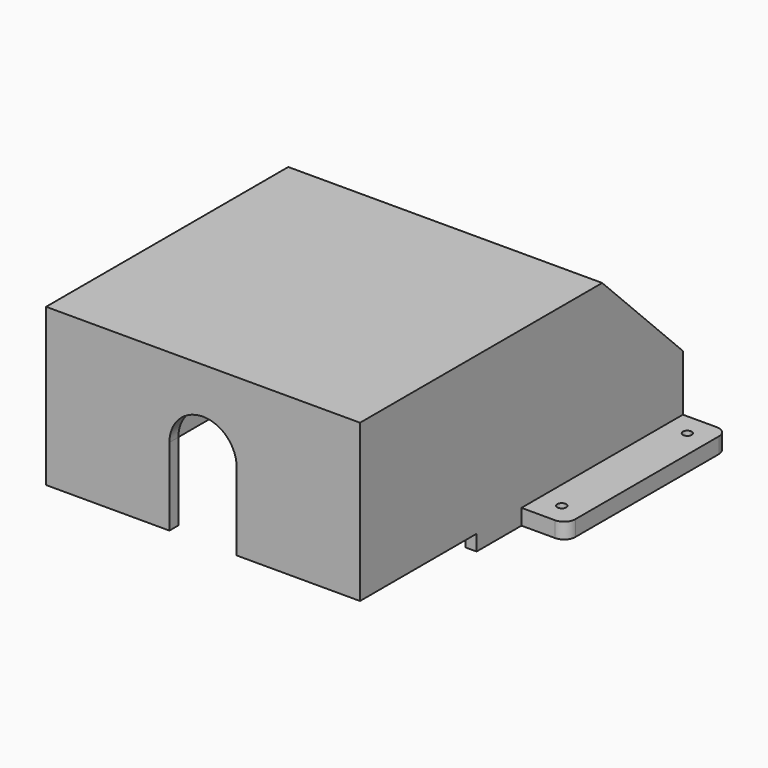
from build123d import *

# Parameters (mm, degrees)
F0_W      = 140
F0_H      = 180
F1_DEPTH  = 70
F2_W      = 130
F2_H      = 170
F3_DEPTH  = 65
F4_SIZE   = 45
F5_W      = 30
F5_H      = 49.6265143156
F6_DEPTH  = 25
F7_R      = 14.99999
F9_DEPTH  = 7
F10_W     = 59.1894394159
F10_H     = 26.9657306075
F11_DEPTH = 25
F12_W     = 90
F12_H     = 7
F13_DEPTH = 20
F14_W     = 90
F14_H     = 7
F15_DEPTH = 20
F17_DEPTH = 25
F19_DEPTH = 25
F20_R     = 5


# Not quite as in the source:
# - a fillet or chamfer is up to 0.001 mm smaller than in the source, because OpenCascade refuses the exact size


with BuildPart() as f1:
    # F0 (on Top) → F1 (new body)
    with BuildSketch(Plane.XY):
        with Locations((46.5964969993, 53.7995101511)):
            Rectangle(F0_W, F0_H)
    extrude(amount=F1_DEPTH)

    # F2 (on face) → F3 (cut)
    with BuildSketch(Plane(origin=(0, 0, 0), x_dir=(1, 0, 0), z_dir=(0, 0, -1))):
        with Locations((46.5964969993, -53.7995101511)):
            Rectangle(F2_W, F2_H)
    extrude(amount=-F3_DEPTH, mode=Mode.SUBTRACT)

    # F4
    f4_edges = [f1.edges().sort_by_distance(p)[0] for p in [
        (46.596497, 143.79951, 70),
        (46.596497, 138.79951, 65),
    ]]
    chamfer(f4_edges, length=F4_SIZE)

    # F5 (on face) → F6 (cut)
    with BuildSketch(Plane.XZ.offset(36.2004898489)):
        with Locations((46.5964969993, 24.8132571578)):
            Rectangle(F5_W, F5_H)
    extrude(amount=-F6_DEPTH, mode=Mode.SUBTRACT)

    # F7 (radius 15 in the source; OpenCascade refuses exactly that, so slightly less here)
    f7_edges = [f1.edges().sort_by_distance(p)[0] for p in [
        (61.596497, -33.70049, 49.626514),
        (31.596497, -33.70049, 49.626514),
    ]]
    fillet(f7_edges, radius=F7_R)

    # F8 (on face) → F9 (join)
    with BuildSketch(Plane(origin=(0, 0, 0), x_dir=(1, 0, 0), z_dir=(0, 0, -1))):
        Polygon((-23.4035030007, -28.7995101511), (-23.4035030007, -143.7995101511), (116.5964969993, -143.7995101511), (116.5964969993, -28.7995101511), (111.5964969993, -28.7995101511), (111.5964969993, -138.7995101511), (-18.4035030007, -138.7995101511), (-18.4035030007, -28.7995101511), align=None)
    extrude(amount=F9_DEPTH)

    # F10 (on face) → F11 (cut)
    with BuildSketch(Plane(origin=(0, 143.7995101511, 0), x_dir=(-1, 0, 0), z_dir=(0, 1, 0))):
        with Locations((-46.5964969993, 6.4828653038)):
            Rectangle(F10_W, F10_H)
    extrude(amount=-F11_DEPTH, mode=Mode.SUBTRACT)

    # F12 (on face) → F13 (join)
    with BuildSketch(Plane(origin=(-23.4035030007, 0, 0), x_dir=(0, -1, 0), z_dir=(-1, 0, 0))):
        with Locations((-98.7995101511, -3.5)):
            Rectangle(F12_W, F12_H)
    extrude(amount=F13_DEPTH)

    # F14 (on face) → F15 (join)
    with BuildSketch(Plane.YZ.offset(116.5964969993)):
        with Locations((98.7995101511, -3.5)):
            Rectangle(F14_W, F14_H)
    extrude(amount=F15_DEPTH)

    # F16 (on face) → F17 (cut)
    with BuildSketch(Plane.XY):
        with BuildLine():
            ThreePointArc((-33.4035030007, 135.7995101511), (-34.8177165631, 132.3852965888), (-31.4035030007, 133.7995101511))
            ThreePointArc((-31.4035030007, 133.7995101511), (-31.9892894384, 135.2137237135), (-33.4035030007, 135.7995101511))
        make_face()
        with BuildLine():
            ThreePointArc((-33.4035030007, 61.7995101511), (-31.9892894384, 62.3852965888), (-31.4035030007, 63.7995101511))
            ThreePointArc((-31.4035030007, 63.7995101511), (-34.8177165631, 65.2137237135), (-33.4035030007, 61.7995101511))
        make_face()
    extrude(amount=-F17_DEPTH, mode=Mode.SUBTRACT)

    # F18 (on face) → F19 (cut)
    with BuildSketch(Plane.XY):
        with BuildLine():
            ThreePointArc((126.5964969993, 61.7995101511), (128.0107105616, 62.3852965888), (128.5964969993, 63.7995101511))
            ThreePointArc((128.5964969993, 63.7995101511), (125.1822834369, 65.2137237135), (126.5964969993, 61.7995101511))
        make_face()
        with BuildLine():
            ThreePointArc((126.5964969993, 135.7995101511), (125.1822834369, 132.3852965888), (128.5964969993, 133.7995101511))
            ThreePointArc((128.5964969993, 133.7995101511), (128.0107105616, 135.2137237135), (126.5964969993, 135.7995101511))
        make_face()
    extrude(amount=-F19_DEPTH, mode=Mode.SUBTRACT)

    # F20
    f20_edges = [f1.edges().sort_by_distance(p)[0] for p in [
        (-43.403503, 53.79951, -3.5),
        (-43.403503, 143.79951, -3.5),
        (136.596497, 143.79951, -3.5),
        (136.596497, 53.79951, -3.5),
    ]]
    fillet(f20_edges, radius=F20_R)


solid = f1.part
